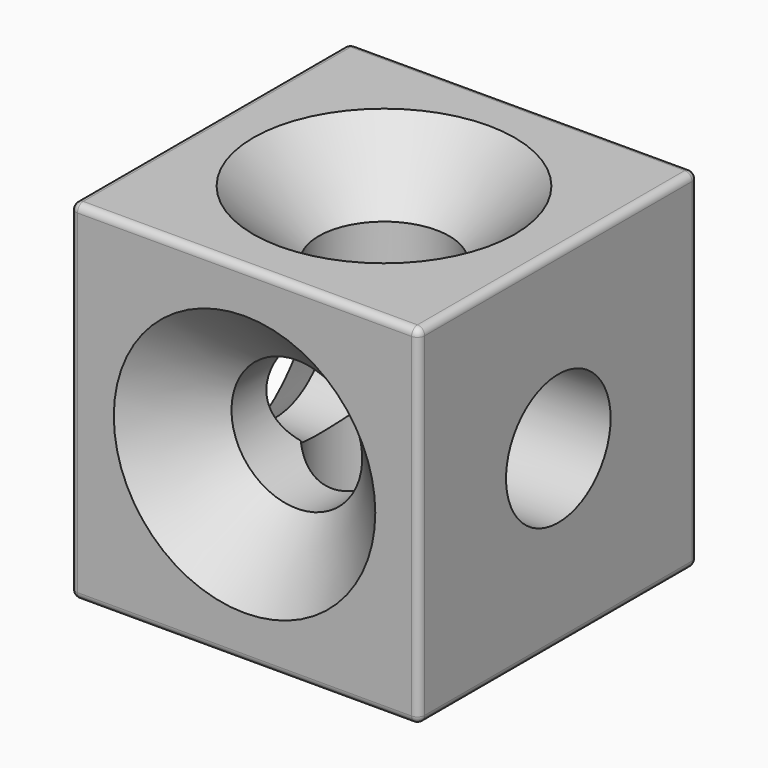
from build123d import *

# Parameters (mm, degrees)
F0_W            = 48
F0_H            = 48
F1_DEPTH        = 48
F2_R            = 1
F3_R            = 1
F4_T1_DEPTH     = 46
F4_T3_DEPTH     = 46
F4_T5_DEPTH     = 46
F4_S9_W         = 1
F4_S9_H         = 1
F4_T10_DEPTH    = 1
F4_S15_W        = 1
F4_S15_H        = 1
F4_T16_DEPTH    = 1
F4_S21_W        = 1
F4_S21_H        = 1
F4_T22_DEPTH    = 1
F4_S27_W        = 1
F4_S27_H        = 1
F4_T28_DEPTH    = 1
F4_T32_ANGLE    = 90
F4_T34_ANGLE    = 90
F6_D            = 18
F6_CSINK_D      = 36
F6_CSINK_ANGLE  = 90
F8_D            = 18
F8_CSINK_D      = 36
F8_CSINK_ANGLE  = 90
F10_D           = 18
F10_CSINK_D     = 36
F10_CSINK_ANGLE = 90


# Not quite as in the source:
# - a fillet or chamfer that OpenCascade refuses, or shapes differently, is made with other operations: its cross-section is extruded or revolved along the edge and cut away or added


with BuildPart() as f1:
    # F0 (on Front) → F1 (new body)
    with BuildSketch(Plane.XZ):
        Rectangle(F0_W, F0_H)
    extrude(amount=F1_DEPTH)

    # F2
    f2_edges = [f1.edges().sort_by_distance(p)[0] for p in [
        (24, -24, 24),
    ]]
    fillet(f2_edges, radius=F2_R)

    # F3
    f3_edges = [f1.edges().sort_by_distance(p)[0] for p in [
        (-24, -24, 24),
        (-0.5, 0, 24),
        (-0.5, -48, 24),
    ]]
    fillet(f3_edges, radius=F3_R)

    # F4: fillet of radius 1 on 8 edges, made by hand

    # F4_s2 → F4_t1 (cut)
    with BuildSketch(Plane.XY.offset(-23)):
        with BuildLine():
            ThreePointArc((-23, -48), (-23.7071067812, -47.7071067812), (-24, -47))
            Line((-24, -47), (-24, -48))
            Line((-24, -48), (-23, -48))
        make_face()
        with BuildLine():
            ThreePointArc((-23, 0), (-23.7071067812, -0.2928932188), (-24, -1))
            Line((-24, -1), (-24, 0))
            Line((-24, 0), (-23, 0))
        make_face()
    extrude(amount=F4_T1_DEPTH, mode=Mode.SUBTRACT)

    # F4_s4 → F4_t3 (cut)
    with BuildSketch(Plane.YZ.offset(-23)):
        with BuildLine():
            ThreePointArc((0, -23), (-0.2928932188, -23.7071067812), (-1, -24))
            Line((-1, -24), (0, -24))
            Line((0, -24), (0, -23))
        make_face()
        with BuildLine():
            ThreePointArc((-48, -23), (-47.7071067812, -23.7071067812), (-47, -24))
            Line((-47, -24), (-48, -24))
            Line((-48, -24), (-48, -23))
        make_face()
    extrude(amount=F4_T3_DEPTH, mode=Mode.SUBTRACT)

    # F4_s6 → F4_t5 (cut)
    with BuildSketch(Plane.XZ.offset(1)):
        with BuildLine():
            ThreePointArc((-24, -23), (-23.7071067812, -23.7071067812), (-23, -24))
            Line((-23, -24), (-24, -24))
            Line((-24, -24), (-24, -23))
        make_face()
        with BuildLine():
            ThreePointArc((24, -23), (23.7071067812, -23.7071067812), (23, -24))
            Line((23, -24), (24, -24))
            Line((24, -24), (24, -23))
        make_face()
    extrude(amount=F4_T5_DEPTH, mode=Mode.SUBTRACT)


with BuildPart() as f4_tool8:
    # F4_s9 → F4_t10 (new body)
    with BuildSketch(Plane.XZ.offset(1)):
        with Locations((-23.5, 23.5)):
            Rectangle(F4_S9_W, F4_S9_H)
    extrude(amount=-F4_T10_DEPTH)

    # F4_s11 → F4_t12 (revolve, cut)
    with BuildSketch(Plane(origin=(-23, -1, 23), x_dir=(0.7071067812, 0, -0.7071067812), z_dir=(0.7071067812, 0, 0.7071067812))):
        with BuildLine():
            ThreePointArc((0, -1), (1, 0), (0, 1))
            Line((0, 1), (0, -1))
        make_face()
    revolve(axis=Axis((-23, -1, 23), (0, 1, 0)), mode=Mode.SUBTRACT)


with BuildPart() as f1_1:
    add(f1.part)

    # F4_t7: cut F4_tool8
    add(f4_tool8.part, mode=Mode.SUBTRACT)


with BuildPart() as f4_tool14:
    # F4_s15 → F4_t16 (new body)
    with BuildSketch(Plane.XZ.offset(47)):
        with Locations((-23.5, 23.5)):
            Rectangle(F4_S15_W, F4_S15_H)
    extrude(amount=F4_T16_DEPTH)

    # F4_s17 → F4_t18 (revolve, cut)
    with BuildSketch(Plane(origin=(-23, -47, 23), x_dir=(0.7071067812, 0, -0.7071067812), z_dir=(-0.7071067812, 0, -0.7071067812))):
        with BuildLine():
            ThreePointArc((0, -1), (1, 0), (0, 1))
            Line((0, 1), (0, -1))
        make_face()
    revolve(axis=Axis((-23, -47, 23), (0, -1, 0)), mode=Mode.SUBTRACT)


with BuildPart() as f1_2:
    add(f1_1.part)

    # F4_t13: cut F4_tool14
    add(f4_tool14.part, mode=Mode.SUBTRACT)


with BuildPart() as f4_tool20:
    # F4_s21 → F4_t22 (new body)
    with BuildSketch(Plane.XZ.offset(47)):
        with Locations((-23.5, -23.5)):
            Rectangle(F4_S21_W, F4_S21_H)
    extrude(amount=F4_T22_DEPTH)

    # F4_s23 → F4_t24 (revolve, cut)
    with BuildSketch(Plane(origin=(-23, -47, -23), x_dir=(0.7071067812, 0, 0.7071067812), z_dir=(0.7071067812, 0, -0.7071067812))):
        with BuildLine():
            ThreePointArc((0, -1), (1, 0), (0, 1))
            Line((0, 1), (0, -1))
        make_face()
    revolve(axis=Axis((-23, -47, -23), (0, -1, 0)), mode=Mode.SUBTRACT)


with BuildPart() as f1_3:
    add(f1_2.part)

    # F4_t19: cut F4_tool20
    add(f4_tool20.part, mode=Mode.SUBTRACT)


with BuildPart() as f4_tool26:
    # F4_s27 → F4_t28 (new body)
    with BuildSketch(Plane.XZ.offset(1)):
        with Locations((-23.5, -23.5)):
            Rectangle(F4_S27_W, F4_S27_H)
    extrude(amount=-F4_T28_DEPTH)

    # F4_s29 → F4_t30 (revolve, cut)
    with BuildSketch(Plane(origin=(-23, -1, -23), x_dir=(0.7071067812, 0, 0.7071067812), z_dir=(-0.7071067812, 0, 0.7071067812))):
        with BuildLine():
            ThreePointArc((0, -1), (1, 0), (0, 1))
            Line((0, 1), (0, -1))
        make_face()
    revolve(axis=Axis((-23, -1, -23), (0, 1, 0)), mode=Mode.SUBTRACT)


with BuildPart() as f1_4:
    add(f1_3.part)

    # F4_t25: cut F4_tool26
    add(f4_tool26.part, mode=Mode.SUBTRACT)

    # F4_s31 → F4_t32 (revolve, cut)
    with BuildSketch(Plane.XZ.offset(1)):
        with BuildLine():
            ThreePointArc((24, -23), (23.7071067812, -23.7071067812), (23, -24))
            Line((23, -24), (24, -24))
            Line((24, -24), (24, -23))
        make_face()
    revolve(axis=Axis((23, -1, -24), (0, 0, 1)), revolution_arc=F4_T32_ANGLE, mode=Mode.SUBTRACT)

    # F4_s33 → F4_t34 (revolve, cut)
    with BuildSketch(Plane.XZ.offset(47)):
        with BuildLine():
            ThreePointArc((24, -23), (23.7071067812, -23.7071067812), (23, -24))
            Line((23, -24), (24, -24))
            Line((24, -24), (24, -23))
        make_face()
    revolve(axis=Axis((23, -47, -24), (0, 0, -1)), revolution_arc=F4_T34_ANGLE, mode=Mode.SUBTRACT)

    # F6 (through all)
    with Locations(Plane.XY.offset(24)):
        with Locations((0, -24)):
            CounterSinkHole(F6_D / 2, F6_CSINK_D / 2, counter_sink_angle=F6_CSINK_ANGLE)

    # F8 (through all)
    with Locations(Plane(origin=(-24, 0, 0), x_dir=(0, -1, 0), z_dir=(-1, 0, 0))):
        with Locations((24, 0)):
            CounterSinkHole(F8_D / 2, F8_CSINK_D / 2, counter_sink_angle=F8_CSINK_ANGLE)

    # F10 (through all)
    with Locations(Plane.XZ.offset(48)):
        with Locations((0, 0)):
            CounterSinkHole(F10_D / 2, F10_CSINK_D / 2, counter_sink_angle=F10_CSINK_ANGLE)


solid = f1_4.part
